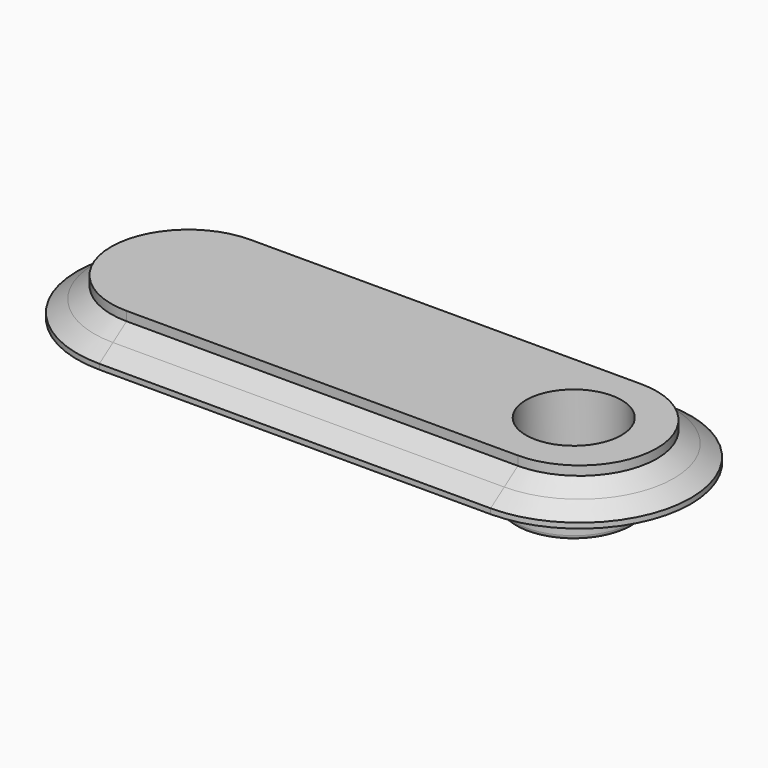
from build123d import *

# Parameters (mm, degrees)
F1_DEPTH         = 1.6
F4_DEPTH         = 1.3
F5_SIZE2         = 1.3
F5_SIZE          = 0.9
F5_2_SIZE2       = 1.29999
F5_2_SIZE        = 0.89999
F6_R             = 4.5
F6_R_2           = 3.26
F7_DEPTH         = 3
F8_DEPTH         = 2.901
F9_R             = 3.645
F9_R_2           = 3.26
F10_DEPTH        = 5
F11_W            = 0.8
F11_H            = 1.2
F13_ANGLE_BACK   = 30
F13_ANGLE        = 60
F13_COPIES_COUNT = 3
F14_ANGLE_BACK   = 15
F14_ANGLE        = 30
F14_COPIES_COUNT = 3
F15_R            = 0.3


# Not quite as in the source:
# - a fillet or chamfer is up to 0.001 mm smaller than in the source, because OpenCascade refuses the exact size
# - after a boolean that leaves OpenCascade's solid faulty, fix() repairs it
# - a pattern or mirror of a feature is missing from the dataset's text; its kind, count and spacing are read off the source's solid


with BuildPart() as f1:
    # F0 (on Top) → F1 (new body)
    with BuildSketch(Plane.XY):
        with BuildLine():
            Line((14.95, 5.9), (-14.95, 5.9))
            ThreePointArc((-14.95, 5.9), (-20.85, 0), (-14.95, -5.9))
            Line((-14.95, -5.9), (14.95, -5.9))
            ThreePointArc((14.95, -5.9), (20.85, 0), (14.95, 5.9))
        make_face()
    extrude(amount=F1_DEPTH)

    # F3 (on offset) → F4 (join)
    with BuildSketch(Plane.XY.offset(-1.3)):
        with BuildLine():
            Line((14.95, 8.5), (-14.95, 8.5))
            ThreePointArc((-14.95, 8.5), (-23.45, 0), (-14.95, -8.5))
            Line((-14.95, -8.5), (14.95, -8.5))
            ThreePointArc((14.95, -8.5), (23.45, 0), (14.95, 8.5))
        make_face()
    extrude(amount=F4_DEPTH)

    # F5
    f5_edges = [f1.edges().sort_by_distance(p)[0] for p in [
        (0, 8.5, 0),
    ]]
    f5_side = f1.faces().sort_by_distance((0, 8.5, -0.65))[0]
    chamfer(f5_edges, length=F5_SIZE, length2=F5_SIZE2, reference=f5_side)

    # F5#2 (size 0.9 and 1.3 in the source; OpenCascade refuses exactly that, so slightly less here)
    f5_2_edges = [f1.edges().sort_by_distance(p)[0] for p in [
        (0, -5.9, 0),
    ]]
    f5_2_side = f1.faces().sort_by_distance((0, -5.9, 0.8))[0]
    chamfer(f5_2_edges, length=F5_2_SIZE, length2=F5_2_SIZE2, reference=f5_2_side)

    # F6 (on face) → F7 (join)
    with BuildSketch(Plane(origin=(0, 0, -1.3), x_dir=(1, 0, 0), z_dir=(0, 0, -1))):
        with Locations((14.5, 0)):
            Circle(F6_R)
        with Locations((14.5, 0)):
            Circle(F6_R_2, mode=Mode.SUBTRACT)
    extrude(amount=F7_DEPTH)

    # F8 (cut, through all): a face of the model
    f8_faces = [f1.faces().sort_by_distance(p)[0] for p in [
        (14.5, 0, -1.3),
    ]]
    extrude(f8_faces, amount=-F8_DEPTH, mode=Mode.SUBTRACT)

    # F9 (on face) → F10 (cut)
    with BuildSketch(Plane.XY.offset(1.6)):
        with Locations((14.5, 0)):
            Circle(F9_R)
        with Locations((14.5, 0)):
            Circle(F9_R_2, mode=Mode.SUBTRACT)
    extrude(amount=-F10_DEPTH, mode=Mode.SUBTRACT)

    # F11 (on Front) → F12 (revolve)
    with BuildSketch(Plane.XZ):
        with Locations((-17.35, -1.9)):
            Rectangle(F11_W, F11_H)
    revolve(axis=Axis((-14.5, 0, 1.6), (0, 0, 1)))

    # F11 (on Front) → F13 (revolve)
    with BuildSketch(Plane.XZ, mode=Mode.PRIVATE) as f13_sk:
        Polygon((-16.95, -4), (-16.95, -2.5), (-17.75, -2.5), (-18.55, -2.5), (-17.75, -4), align=None)
    f13 = revolve(f13_sk.sketch.rotate(Axis((-14.5, 0, 1.6), (0, 0, 1)), -F13_ANGLE_BACK), axis=Axis((-14.5, 0, 1.6), (0, 0, 1)), revolution_arc=F13_ANGLE)

    # F13_copies: F13 ×3 about axis
    f13_copies_axis = Axis((-14.5, 0, 0), (0, 0, 1))
    for i in range(1, F13_COPIES_COUNT):
        add(f13.rotate(f13_copies_axis, i * 360 / F13_COPIES_COUNT))

    # F11 (on Front) → F14 (revolve)
    with BuildSketch(Plane.XZ, mode=Mode.PRIVATE) as f14_sk:
        Polygon((-16.15, -1.3), (-16.95, -1.3), (-16.95, -2.5), align=None)
    f14 = revolve(f14_sk.sketch.rotate(Axis((-14.5, 0, 1.6), (0, 0, 1)), -F14_ANGLE_BACK), axis=Axis((-14.5, 0, 1.6), (0, 0, 1)), revolution_arc=F14_ANGLE)

    # F14_copies: F14 ×3 about axis
    f14_copies_axis = Axis((-14.5, 0, 0), (0, 0, 1))
    for i in range(1, F14_COPIES_COUNT):
        add(f14.rotate(f14_copies_axis, i * 360 / F14_COPIES_COUNT))

    add(f1.part.fix(), mode=Mode.REPLACE)

    # F15
    f15_edges = [f1.edges().sort_by_distance(p)[0] for p in [
        (10, 0, -4.3),
    ]]
    fillet(f15_edges, radius=F15_R)


solid = f1.part
